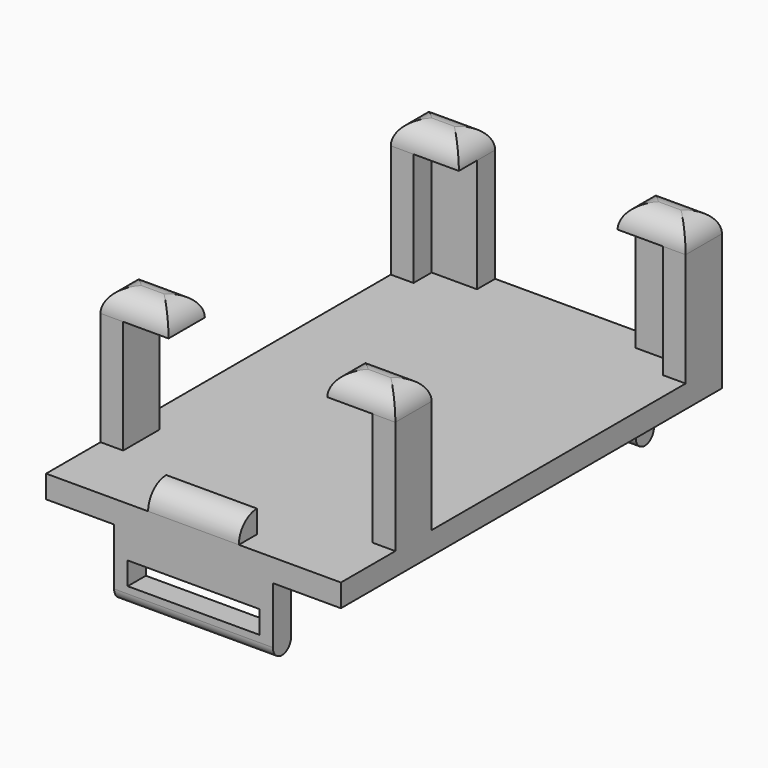
from build123d import *

# Parameters (mm, degrees)
F0_W      = 65
F0_H      = 105
F2_DEPTH  = 5
F3_DEPTH  = 35
F4_W      = 5
F4_H      = 5
F5_DEPTH  = 5
F6_W      = 5
F6_H      = 5
F7_DEPTH  = 5
F8_W      = 5
F8_H      = 10
F9_DEPTH  = 30
F11_W     = 10
F11_H     = 5
F12_DEPTH = 10
F10_W     = 10
F10_H     = 5
F13_DEPTH = 10
F14_DEPTH = 5
F15_DEPTH = 5
F16_W     = 20
F16_H     = 5
F17_DEPTH = 5
F18_W     = 35
F18_H     = 5
F19_DEPTH = 15
F21_W     = 29
F21_H     = 5
F22_DEPTH = 25
F20_W     = 29
F20_H     = 5
F23_DEPTH = 25
F24_R     = 2.49999
F25_R     = 4.99999


# Not quite as in the source:
# - a fillet or chamfer is up to 0.001 mm smaller than in the source, because OpenCascade refuses the exact size


with BuildPart() as f2:
    # F0 (on Top) → F2 (new body)
    with BuildSketch(Plane.XY):
        Rectangle(F0_W, F0_H)
    extrude(amount=F2_DEPTH)

    # F1 (on face) → F3 (join)
    with BuildSketch(Plane.XY):
        Polygon((-22.5, 52.5), (-27.5, 52.5), (-32.5, 52.5), (-32.5, 47.5), (-32.5, 42.5), (-27.5, 42.5), (-27.5, 47.5), (-22.5, 47.5), align=None)
        Polygon((27.5, 52.5), (22.5, 52.5), (22.5, 47.5), (27.5, 47.5), (27.5, 42.5), (32.5, 42.5), (32.5, 52.5), align=None)
    extrude(amount=F3_DEPTH)

    # F4 (on face) → F5 (join)
    with BuildSketch(Plane(origin=(27.5, 0, 0), x_dir=(0, -1, 0), z_dir=(-1, 0, 0))):
        with Locations((-45, 32.5)):
            Rectangle(F4_W, F4_H)
    extrude(amount=F5_DEPTH)

    # F6 (on face) → F7 (join)
    with BuildSketch(Plane.YZ.offset(-27.5)):
        with Locations((45, 32.5)):
            Rectangle(F6_W, F6_H)
    extrude(amount=F7_DEPTH)

    # F8 (on face) → F9 (join)
    with BuildSketch(Plane.XY.offset(5)):
        with Locations((30, -32.5)):
            Rectangle(F8_W, F8_H)
        with Locations((-30, -32.5)):
            Rectangle(F8_W, F8_H)
    extrude(amount=F9_DEPTH)

    # F11 (on face) → F12 (join)
    with BuildSketch(Plane(origin=(27.5, 0, 0), x_dir=(0, -1, 0), z_dir=(-1, 0, 0))):
        with Locations((32.5, 32.5)):
            Rectangle(F11_W, F11_H)
    extrude(amount=F12_DEPTH)

    # F10 (on face) → F13 (join)
    with BuildSketch(Plane.YZ.offset(-27.5)):
        with Locations((-32.5, 32.5)):
            Rectangle(F10_W, F10_H)
    extrude(amount=F13_DEPTH)

    # F14 (add): a face of the model
    f14_faces = [f2.faces().sort_by_distance(p)[0] for p in [
        (22.5, 49.2857142857, 21.7857142857),
    ]]
    extrude(f14_faces, amount=F14_DEPTH)

    # F15 (add): a face of the model
    f15_faces = [f2.faces().sort_by_distance(p)[0] for p in [
        (-22.5, 49.2857142857, 21.7857142857),
    ]]
    extrude(f15_faces, amount=F15_DEPTH)

    # F16 (on face) → F17 (join)
    with BuildSketch(Plane.XY.offset(5)):
        with Locations((0, -50)):
            Rectangle(F16_W, F16_H)
    extrude(amount=F17_DEPTH)

    # F18 (on face) → F19 (join)
    with BuildSketch(Plane(origin=(0, 0, 0), x_dir=(1, 0, 0), z_dir=(0, 0, -1))):
        with Locations((0, 50)):
            Rectangle(F18_W, F18_H)
        with Locations((0, -50)):
            Rectangle(F18_W, F18_H)
    extrude(amount=F19_DEPTH)

    # F21 (on face) → F22 (cut)
    with BuildSketch(Plane.XZ.offset(-47.5)):
        with Locations((0, -8.5)):
            Rectangle(F21_W, F21_H)
    extrude(amount=-F22_DEPTH, mode=Mode.SUBTRACT)

    # F20 (on face) → F23 (cut)
    with BuildSketch(Plane(origin=(0, -47.5, 0), x_dir=(-1, 0, 0), z_dir=(0, 1, 0))):
        with Locations((0, -8.5)):
            Rectangle(F20_W, F20_H)
    extrude(amount=-F23_DEPTH, mode=Mode.SUBTRACT)

    # F24 (radius 2.5 in the source; OpenCascade refuses exactly that, so slightly less here)
    f24_edges = [f2.edges().sort_by_distance(p)[0] for p in [
        (0, 52.5, -15),
        (0, 47.5, -15),
        (0, -52.5, -15),
        (0, -47.5, -15),
    ]]
    fillet(f24_edges, radius=F24_R)

    # F25 (radius 5 in the source; OpenCascade refuses exactly that, so slightly less here)
    f25_edges = [f2.edges().sort_by_distance(p)[0] for p in [
        (-32.5, -32.5, 35),
        (32.5, -32.5, 35),
        (17.5, -32.5, 35),
        (-17.5, -32.5, 35),
        (-25, 52.5, 35),
        (25, 52.5, 35),
        (32.5, 47.5, 35),
        (25, 42.5, 35),
        (17.5, 47.5, 35),
        (-25, 42.5, 35),
        (-17.5, 47.5, 35),
        (-32.5, 47.5, 35),
        (-25, -37.5, 35),
        (-25, -27.5, 35),
        (25, -37.5, 35),
        (25, -27.5, 35),
        (0, -52.5, 10),
    ]]
    fillet(f25_edges, radius=F25_R)


solid = f2.part
